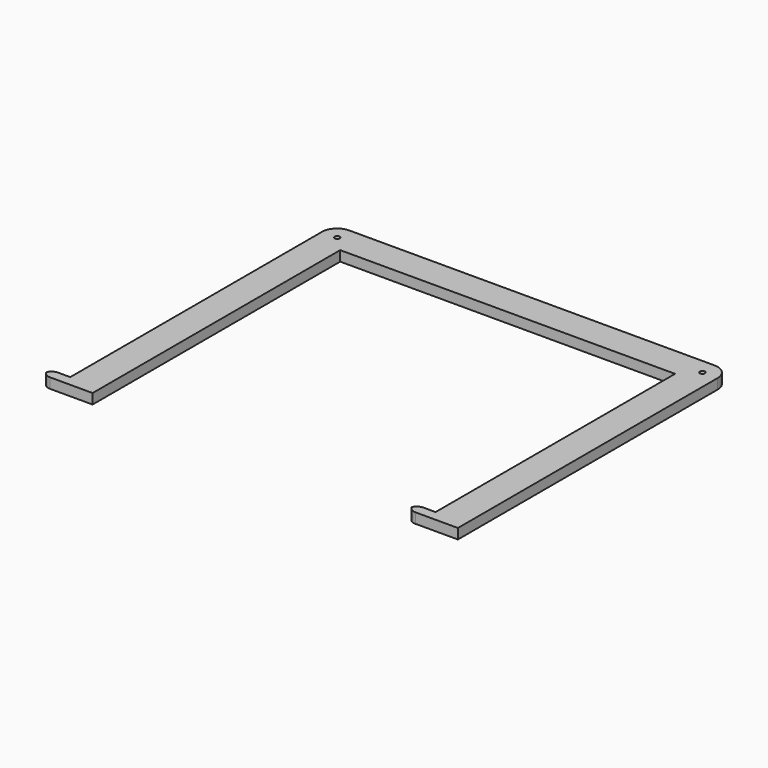
from build123d import *

# Parameters (mm, degrees)
F0_W        = 12.7
F0_H        = 6.35
F0_W_2      = 19.05
F0_H_2      = 187.325
F0_H_3      = 19.05
F0_R        = 1.5875
F0_W_3      = 209.55
F1_DEPTH    = 6.35
F2_R        = 9.525
F3_T1_DEPTH = 31.75


# Not quite as in the source:
# - a fillet or chamfer that OpenCascade refuses, or shapes differently, is made with other operations: its cross-section is extruded or revolved along the edge and cut away or added
# - a length typed as a fraction of an inch, garbled in the dataset ("3 / 203.2 mm" for 3/8 in), is restored


with BuildPart() as f1:
    # F0 (on Top) → F1 (new body)
    with BuildSketch(Plane.XY):
        with Locations((-254, -190.5)):
            Rectangle(F0_W, F0_H)
        with Locations((-238.125, -190.5)):
            Rectangle(F0_W_2, F0_H)
        with Locations((-238.125, -93.6625)):
            Rectangle(F0_W_2, F0_H_2)
        with Locations((-238.125, 9.525)):
            Rectangle(F0_W_2, F0_H_3)
        with Locations((-238.125, 9.525)):
            Circle(F0_R, mode=Mode.SUBTRACT)
        with Locations((-123.825, 9.525)):
            Rectangle(F0_W_3, F0_H_3)
        with Locations((-9.525, 9.525)):
            Rectangle(F0_W_2, F0_H_3)
        with Locations((-9.525, 9.525)):
            Circle(F0_R, mode=Mode.SUBTRACT)
        with Locations((-9.525, -93.6625)):
            Rectangle(F0_W_2, F0_H_2)
        with Locations((-9.525, -190.5)):
            Rectangle(F0_W_2, F0_H)
        with Locations((-25.4, -190.5)):
            Rectangle(F0_W, F0_H)
    extrude(amount=F1_DEPTH)

    # F2
    f2_edges = [f1.edges().sort_by_distance(p)[0] for p in [
        (0, 19.05, 3.175),
        (-247.65, 19.05, 3.175),
    ]]
    fillet(f2_edges, radius=F2_R)

    # F3: fillet of radius 5.08 on 4 edges, made by hand

    # F3_s2 → F3_t1 (cut)
    with BuildSketch(Plane.XY.offset(-12.7)):
        with BuildLine():
            ThreePointArc((-255.27, -187.325), (-258.8621024484, -188.8128975516), (-260.35, -192.405))
            Line((-260.35, -192.405), (-260.35, -187.325))
            Line((-260.35, -187.325), (-255.27, -187.325))
        make_face()
        with BuildLine():
            ThreePointArc((-31.75, -192.405), (-30.2621024484, -188.8128975516), (-26.67, -187.325))
            Line((-26.67, -187.325), (-31.75, -187.325))
            Line((-31.75, -187.325), (-31.75, -192.405))
        make_face()
        with BuildLine():
            ThreePointArc((-260.35, -188.595), (-258.8621024484, -192.1871024484), (-255.27, -193.675))
            Line((-255.27, -193.675), (-260.35, -193.675))
            Line((-260.35, -193.675), (-260.35, -188.595))
        make_face()
        with BuildLine():
            ThreePointArc((-26.67, -193.675), (-30.2621024484, -192.1871024484), (-31.75, -188.595))
            Line((-31.75, -188.595), (-31.75, -193.675))
            Line((-31.75, -193.675), (-26.67, -193.675))
        make_face()
    extrude(amount=F3_T1_DEPTH, mode=Mode.SUBTRACT)


solid = f1.part
